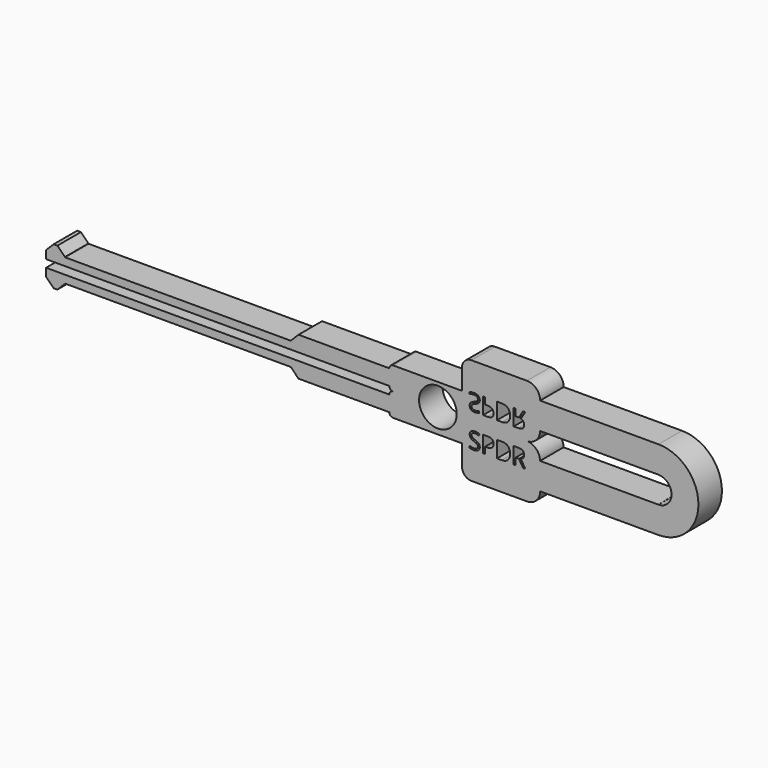
from build123d import *

# Parameters (mm, degrees)
F1_DEPTH      = 19.812
F2_TEXT_SIZE  = 15.49289025
F3_DEPTH      = 19.813
F5_DEPTH      = 231.394
F6_W          = 152.4
F6_H          = 5.2504474509
F7_DEPTH      = 25.4
F8_R          = 12.7
F9_DEPTH      = 93.472
F10_T1_DEPTH  = 45.9402991577
F10_T6_DEPTH  = 31.3787466087
F10_T11_DEPTH = 31.3787466087
F11_DEPTH     = 79.756
F13_DEPTH     = 19.812


# Not quite as in the source:
# - a fillet or chamfer that OpenCascade refuses, or shapes differently, is made with other operations: its cross-section is extruded or revolved along the edge and cut away or added
# - Text() gives the source's letters only with a copy of the font that has no kerning and outlines rounded to 1/6400 em; it was checked with that copy


with BuildPart() as f1:
    # F0 (on Front) → F1 (new body)
    with BuildSketch(Plane.XZ):
        with BuildLine():
            Line((41.91, 7.7904474509), (-48.26, 7.7904474509))
            ThreePointArc((-48.26, 7.7904474509), (-50.0560512242, 7.0464986751), (-50.8, 5.2504474509))
            Line((-50.8, 5.2504474509), (-50.8, -5.2504474509))
            ThreePointArc((-50.8, -5.2504474509), (-50.0560512242, -7.0464986751), (-48.26, -7.7904474509))
            Line((-48.26, -7.7904474509), (-1.8003238863, -7.7904474509))
            Line((-1.8003238863, -7.7904474509), (50.8, -7.7904474509))
            Line((50.8, -7.7904474509), (50.8, -1.0995525491))
            ThreePointArc((50.8, -1.0995525491), (48.1961792847, 5.1866267357), (41.91, 7.7904474509))
        make_face()
        with BuildLine():
            Line((50.8811640834, -7.7904474509), (50.8, -7.7904474509))
            Line((50.8, -7.7904474509), (-1.8003238863, -7.7904474509))
            Line((-1.8003238863, -7.7904474509), (-1.8003238863, -21.6758669489))
            ThreePointArc((-1.8003238863, -21.6758669489), (0.0595480531, -26.1659950094), (4.5496761137, -28.0258669489))
            Line((4.5496761137, -28.0258669489), (41.9911640834, -28.0258669489))
            ThreePointArc((41.9911640834, -28.0258669489), (48.2773433682, -25.4220462336), (50.8811640834, -19.1358669489))
            Line((50.8811640834, -19.1358669489), (50.8811640834, -7.7904474509))
        make_face()
    extrude(amount=-F1_DEPTH)

    # F2 (on face) → F3 (cut, through all)
    with BuildSketch(Plane.XZ):
        with BuildLine():
            add(Edge.make_bspline(
                [(28.0818086154, -6.8385909305), (29.240144238, -5.706883713), (29.240144238, -3.49188456)],
                knots=[0, 0, 0, 1, 1, 1], degree=2))
            add(Edge.make_bspline(
                [(29.240144238, -3.49188456), (29.240144238, -1.3277214532), (28.1544315384, -0.2311153152)],
                knots=[0, 0, 0, 1, 1, 1], degree=2))
            add(Edge.make_bspline(
                [(28.1544315384, -0.2311153152), (27.0687188389, 0.8654908228), (24.926342609, 0.8654908228)],
                knots=[0, 0, 0, 1, 1, 1], degree=2))
            Line((24.926342609, 0.8654908228), (23.0575127226, 0.8654908228))
            Line((23.0575127226, 0.8654908228), (23.0575127226, -7.9702981479))
            Line((23.0575127226, -7.9702981479), (24.6237470963, -7.9702981479))
            add(Edge.make_bspline(
                [(24.6237470963, -7.9702981479), (26.9234729928, -7.9702981479), (28.0818086154, -6.8385909305)],
                knots=[0, 0, 0, 1, 1, 1], degree=2))
        make_face()
        with Locations((2.4204987567, -9.0814288706)):
            Text('SPDR', F2_TEXT_SIZE, font='Open Sans', text_align=(TextAlign.LEFT, TextAlign.BOTTOM))
        with BuildLine():
            Line((13.7303086392, 0.8654908228), (13.7303086392, -3.6274473497))
            Line((13.7303086392, -3.6274473497), (14.8898546439, -3.6274473497))
            add(Edge.make_bspline(
                [(14.8898546439, -3.6274473497), (16.5989140996, -3.6274473497), (17.3626651736, -3.0755131346)],
                knots=[0, 0, 0, 1, 1, 1], degree=2))
            add(Edge.make_bspline(
                [(17.3626651736, -3.0755131346), (18.1264162477, -2.5235789194), (18.1264162477, -1.3035138122)],
                knots=[0, 0, 0, 1, 1, 1], degree=2))
            add(Edge.make_bspline(
                [(18.1264162477, -1.3035138122), (18.1264162477, -0.2069076742), (17.4074493095, 0.3292915743)],
                knots=[0, 0, 0, 1, 1, 1], degree=2))
            add(Edge.make_bspline(
                [(17.4074493095, 0.3292915743), (16.6884823713, 0.8654908228), (15.1682425156, 0.8654908228)],
                knots=[0, 0, 0, 1, 1, 1], degree=2))
            Line((15.1682425156, 0.8654908228), (13.7303086392, 0.8654908228))
        make_face()
        with BuildLine():
            Line((34.3527980205, 0.8509662382), (34.3527980205, -3.3781086473))
            Line((34.3527980205, -3.3781086473), (36.1175350505, -3.3781086473))
            add(Edge.make_bspline(
                [(36.1175350505, -3.3781086473), (37.4780044756, -3.3781086473), (38.1134550523, -2.8370678706)],
                knots=[0, 0, 0, 1, 1, 1], degree=2))
            add(Edge.make_bspline(
                [(38.1134550523, -2.8370678706), (38.7489056289, -2.2960270939), (38.7489056289, -1.2139455405)],
                knots=[0, 0, 0, 1, 1, 1], degree=2))
            add(Edge.make_bspline(
                [(38.7489056289, -1.2139455405), (38.7489056289, -0.1173394024), (38.1025616138, 0.3668134179)],
                knots=[0, 0, 0, 1, 1, 1], degree=2))
            add(Edge.make_bspline(
                [(38.1025616138, 0.3668134179), (37.4562175987, 0.8509662382), (36.0255460147, 0.8509662382)],
                knots=[0, 0, 0, 1, 1, 1], degree=2))
            Line((36.0255460147, 0.8509662382), (34.3527980205, 0.8509662382))
        make_face()
    extrude(amount=-F3_DEPTH, mode=Mode.SUBTRACT)

    # F4: F1 across face


with BuildPart() as f1_1:
    add(f1.part)
    add(f1.part.mirror(Plane(origin=(-3.175, 9.906, 7.7904474509), x_dir=(1, 0, 0), z_dir=(0, 0, 1))))

    # F5 (add): faces of the model
    f5_faces = [f1_1.faces().sort_by_distance(p)[0] for p in [
        (-50.8, 9.906, 15.5808949019),
        (-50.8, 9.906, 0),
    ]]
    extrude(f5_faces, amount=F5_DEPTH)

    # F6 (on face) → F7 (cut)
    with BuildSketch(Plane.XZ):
        with Locations((-193.294, -7.8756711764)):
            Rectangle(F6_W, F6_H)
        with Locations((-193.294, -2.6252237255)):
            Rectangle(F6_W, F6_H)
        with Locations((-193.294, 23.4565660783)):
            Rectangle(F6_W, F6_H)
        with Locations((-193.294, 18.2061186273)):
            Rectangle(F6_W, F6_H)
    extrude(amount=-F7_DEPTH, mode=Mode.SUBTRACT)

    # F8 (on face) → F9 (cut)
    with BuildSketch(Plane(origin=(0, 19.812, 0), x_dir=(-1, 0, 0), z_dir=(0, 1, 0))):
        with Locations((18.0597826838, 8.4171891212)):
            Circle(F8_R)
    extrude(amount=-F9_DEPTH, mode=Mode.SUBTRACT)

    # F10: chamfer of 5.08 on 8 edges, made by hand

    # F10_s2 → F10_t1 (cut)
    with BuildSketch(Plane.XZ.offset(-32.8761495789)):
        Polygon((-112.014, -5.2504474509), (-117.094, -0.1704474509), (-117.094, -5.2504474509), align=None)
        Polygon((-269.494, -0.1704474509), (-274.574, -5.2504474509), (-269.494, -5.2504474509), align=None)
        Polygon((-277.114, -5.2504474509), (-282.194, -0.1704474509), (-282.194, -5.2504474509), align=None)
        Polygon((-112.014, 20.8313423528), (-117.094, 15.7513423528), (-117.094, 20.8313423528), align=None)
        Polygon((-269.494, 15.7513423528), (-274.574, 20.8313423528), (-269.494, 20.8313423528), align=None)
        Polygon((-277.114, 20.8313423528), (-282.194, 15.7513423528), (-282.194, 20.8313423528), align=None)
    extrude(amount=F10_T1_DEPTH, mode=Mode.SUBTRACT)


with BuildPart() as f10_tool4:
    # F10_s5 → F10_t6 (new body)
    with BuildSketch(Plane.XY.offset(2.516745323)):
        Polygon((-112.014, 0), (-117.094, 5.08), (-117.094, 0), align=None)
    extrude(amount=F10_T6_DEPTH)

    split(bisect_by=Plane(origin=(-66.4226711764, 0, 66.4226711764), x_dir=(0, 1, 0), z_dir=(-0.7071067812, 0, 0.7071067812)), keep=Keep.TOP)


with BuildPart() as f1_2:
    add(f1_1.part)

    # F10_t3: cut F10_tool4
    add(f10_tool4.part, mode=Mode.SUBTRACT)


with BuildPart() as f10_tool9:
    # F10_s10 → F10_t11 (new body)
    with BuildSketch(Plane.XY.offset(33.8954919317)):
        Polygon((-274.574, 0), (-269.494, 5.08), (-269.494, 0), align=None)
    extrude(amount=-F10_T11_DEPTH)

    split(bisect_by=Plane(origin=(-126.8713288236, 0, -126.8713288236), x_dir=(0, 1, 0), z_dir=(0.7071067812, 0, 0.7071067812)), keep=Keep.TOP)


with BuildPart() as f1_3:
    add(f1_2.part)

    # F10_t8: cut F10_tool9
    add(f10_tool9.part, mode=Mode.SUBTRACT)

    # F11 (add): faces of the model
    f11_faces = [f1_3.faces().sort_by_distance(p)[0] for p in [
        (50.8811640834, 9.906, 29.0440521018),
        (50.8, 9.906, 20.0258949019),
        (50.8, 9.906, -4.445),
        (50.8811640834, 9.906, -13.4631571999),
    ]]
    extrude(f11_faces, amount=F11_DEPTH)

    # F12 (on face) → F13 (join, through all)
    with BuildSketch(Plane(origin=(0, 19.812, 0), x_dir=(-1, 0, 0), z_dir=(0, 1, 0))):
        with BuildLine():
            Line((-130.6371640834, 23.3713423528), (-130.6371640834, 34.7167618508))
            ThreePointArc((-130.6371640834, 34.7167618508), (-157.5634784833, 7.7904474509), (-130.6371640834, -19.1358669489))
            Line((-130.6371640834, -19.1358669489), (-130.6371640834, -7.7904474509))
            Line((-130.6371640834, -7.7904474509), (-130.6371640834, -1.0991820347))
            ThreePointArc((-130.6371640834, -1.0991820347), (-139.446, 7.7904474509), (-130.6371640834, 16.6800769365))
            Line((-130.6371640834, 16.6800769365), (-130.6371640834, 23.3713423528))
        make_face()
    extrude(amount=-F13_DEPTH)


solid = f1_3.part
